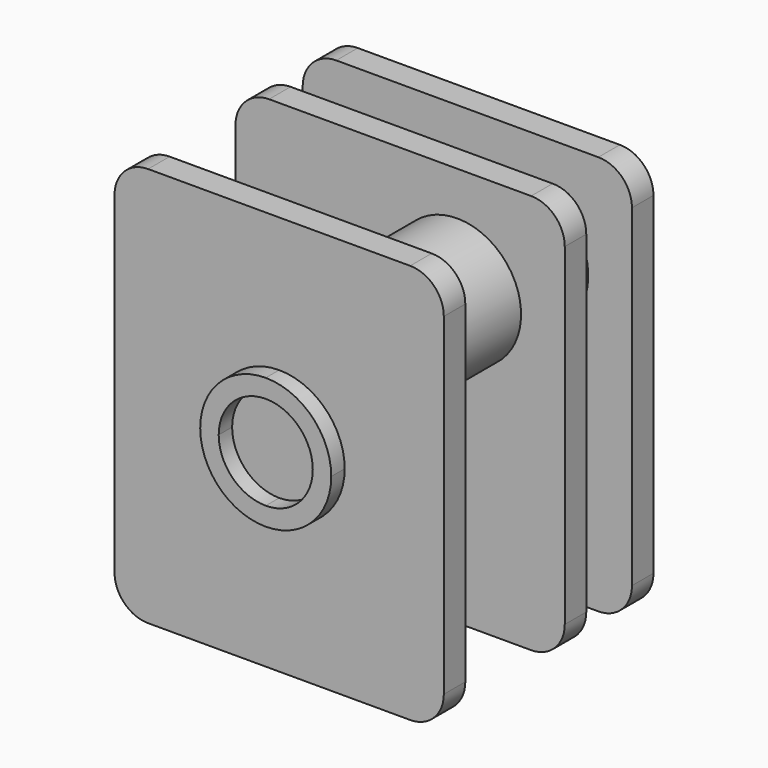
from build123d import *

# Parameters (mm, degrees)
F0_W      = 9.8
F0_H      = 11.9
F1_DEPTH  = 0.8
F2_R      = 1.9
F4_DEPTH  = 6.9
F3_R      = 1.9
F5_DEPTH  = 7.7
F6_W      = 9.8
F6_H      = 0.5256494999
F7_DEPTH  = 25.4
F8_W      = 9.8
F8_H      = 0.8
F9_DEPTH  = 11.37412
F10_DEPTH = 25.4
F11_R     = 1
F13_DEPTH = 0.5


with BuildPart() as f1:
    # F0 (on Front) → F1 (new body)
    with BuildSketch(Plane.XZ):
        Rectangle(F0_W, F0_H)
    extrude(amount=F1_DEPTH)

    # F2 (on face) → F4 (join)
    with BuildSketch(Plane.XZ.offset(0.8)):
        with Locations((-1.7, -2.75)):
            Circle(F2_R)
    extrude(amount=F4_DEPTH)

    # F3 (on face) → F5 (join)
    with BuildSketch(Plane(origin=(0, 0, 0), x_dir=(-1, 0, 0), z_dir=(0, 1, 0))):
        with Locations((-1.69952, 2.74952)):
            Circle(F3_R)
    extrude(amount=-F5_DEPTH)

    # F6 (on face) → F7 (join)
    with BuildSketch(Plane.XZ.offset(0.8)):
        with Locations((0, -5.6871752501)):
            Rectangle(F6_W, F6_H)
    extrude(amount=F7_DEPTH)

    # F8 (on face) → F9 (join)
    with BuildSketch(Plane.XY.offset(-5.4243505001)):
        with Locations((0, -2.9)):
            Rectangle(F8_W, F8_H)
        with Locations((0, -7.4)):
            Rectangle(F8_W, F8_H)
    extrude(amount=F9_DEPTH)

    # F10 (cut): faces of the model
    f10_faces = [f1.faces().sort_by_distance(p)[0] for p in [
        (0, -17, -5.4243505001),
        (0, -5.15, -5.4243505001),
        (0, -1.65, -5.4243505001),
    ]]
    extrude(f10_faces, amount=-F10_DEPTH, mode=Mode.SUBTRACT)

    # F11
    f11_edges = [f1.edges().sort_by_distance(p)[0] for p in [
        (-4.9, -7.4, 5.949769),
        (-4.9, -2.9, 5.949769),
        (-4.9, -0.4, 5.95),
        (-4.9, -0.4, -5.95),
        (-4.9, -2.9, -5.95),
        (-4.9, -7.4, -5.95),
        (4.9, -7.4, 5.949769),
        (4.9, -2.9, 5.949769),
        (4.9, -0.4, 5.95),
        (4.9, -0.4, -5.95),
        (4.9, -7.4, -5.95),
        (4.9, -2.9, -5.95),
    ]]
    fillet(f11_edges, radius=F11_R)

    # F12 (on face) → F13 (join)
    with BuildSketch(Plane.XZ.offset(7.8)):
        with BuildLine():
            ThreePointArc((0, 1.95), (-1.3788989698, 1.3788174757), (-1.9499999966, -0.0001152501))
            Line((-1.9499999966, -0.0001152501), (-1.3999999953, -0.0001152501))
            ThreePointArc((-1.3999999953, -0.0001152501), (-0.9899902399, 0.9899087458), (0, 1.4))
            Line((0, 1.4), (0, 1.95))
        make_face()
        with BuildLine():
            Line((-1.3999999953, -0.0001152501), (-1.9499999966, -0.0001152501))
            ThreePointArc((-1.9499999966, -0.0001152501), (-1.3788174757, -1.3788989698), (0, -1.95))
            Line((0, -1.95), (0, -1.4))
            ThreePointArc((0, -1.4), (-0.9899087458, -0.9899902399), (-1.3999999953, -0.0001152501))
        make_face()
        with BuildLine():
            ThreePointArc((1.95, 0), (1.3788582233, 1.3788582233), (0, 1.95))
            Line((0, 1.95), (0, 1.4))
            ThreePointArc((0, 1.4), (0.9899494937, 0.9899494937), (1.4, 0))
            ThreePointArc((1.4, 0), (1.3999999988, -5.7625e-05), (1.3999999953, -0.0001152501))
            Line((1.3999999953, -0.0001152501), (1.9499999966, -0.0001152501))
            ThreePointArc((1.9499999966, -0.0001152501), (1.9499999991, -5.7625e-05), (1.95, 0))
        make_face()
        with BuildLine():
            Line((0, -1.4), (0, -1.95))
            ThreePointArc((0, -1.95), (1.3788174757, -1.3788989698), (1.9499999966, -0.0001152501))
            Line((1.9499999966, -0.0001152501), (1.3999999953, -0.0001152501))
            ThreePointArc((1.3999999953, -0.0001152501), (0.9899087458, -0.9899902399), (0, -1.4))
        make_face()
    extrude(amount=F13_DEPTH)


solid = f1.part
